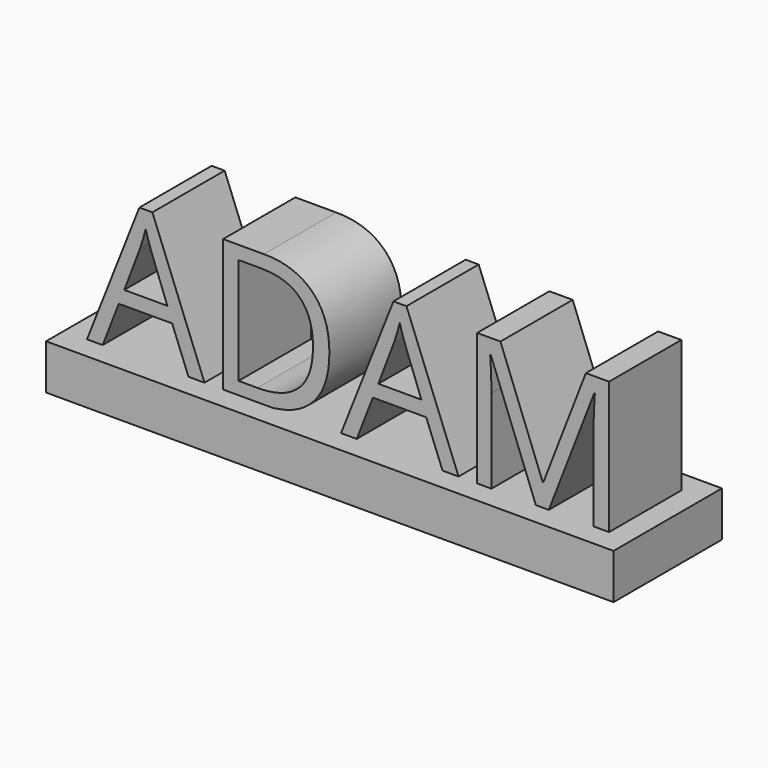
from build123d import *

# Parameters (mm, degrees)
F0_TEXT_SIZE  = 52.4629855944
F1_DEPTH      = 25.4
F2_W          = 159.5881657222
F2_H          = 12.7
F3_DEPTH      = 31.75
F3_DEPTH_BACK = 6.35


# Not quite as in the source:
# - Text() gives the source's letters only with a copy of the font that has no kerning and outlines rounded to 1/6400 em; it was checked with that copy


with BuildPart() as f1:
    # F0 (on Front) → F1 (new body)
    with BuildSketch(Plane.XZ):
        with Locations((3.3994e-06, -0.1952362509)):
            Text('ADAM', F0_TEXT_SIZE, font='Open Sans', text_align=(TextAlign.LEFT, TextAlign.BOTTOM))
    extrude(amount=F1_DEPTH)


with BuildPart() as f3:
    # F2 (on Front) → F3 (new body, two sides)
    with BuildSketch(Plane.XZ) as f3_sk:
        with Locations((73.4440828611, -6.35)):
            Rectangle(F2_W, F2_H)
    extrude(amount=F3_DEPTH)
    extrude(f3_sk.sketch, amount=-F3_DEPTH_BACK)


solid = Compound([f1.part, f3.part])
